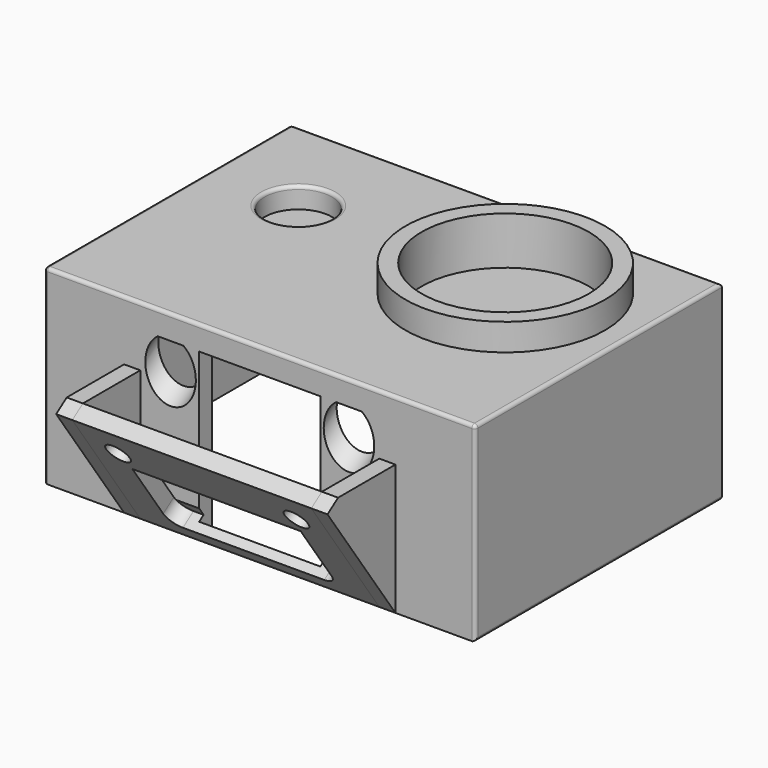
from build123d import *

# Parameters (mm, degrees)
F5_W         = 64
F5_H         = 45.8
F5_W_2       = 59.2
F5_H_2       = 41
F6_DEPTH     = 24.7
F7_W         = 64
F7_H         = 45.8
F7_W_2       = 59.2
F7_H_2       = 41
F8_DEPTH     = 3.6
F9_R         = 5
F10_DEPTH    = 3.1
F11_R        = 14.82
F11_R_2      = 12.42
F12_DEPTH    = 4
F13_DEPTH    = 3.1
F14_R        = 5
F15_DEPTH    = 2.4
F17_R        = 1.75
F18_DEPTH    = 2.4
F20_DEPTH    = 2.4
F22_DEPTH    = 2.4
F23_R        = 1.75
F24_REACH    = 60.9944299909
F25_R        = 0.5
F26_W        = 18
F26_H        = 2.4
F27_DEPTH    = 24.7
F28_R        = 3.75
F29_REACH    = 64.2512842404
F31_DEPTH    = 2.4
F32_T1_DEPTH = 2.4


# Not quite as in the source:
# - a fillet or chamfer that OpenCascade refuses, or shapes differently, is made with other operations: its cross-section is extruded or revolved along the edge and cut away or added
# - a feature names something its author has since deleted; it is built from what else it names


with BuildPart() as f6:
    # F5 (on Top) → F6 (new body)
    with BuildSketch(Plane.XY):
        Rectangle(F5_W, F5_H)
        Rectangle(F5_W_2, F5_H_2, mode=Mode.SUBTRACT)
    extrude(amount=F6_DEPTH)

    # F7 (on face) → F8 (join)
    with BuildSketch(Plane.XY.offset(24.7)):
        Rectangle(F7_W, F7_H)
        Rectangle(F7_W_2, F7_H_2, mode=Mode.SUBTRACT)
        Rectangle(F7_W_2, F7_H_2)
    extrude(amount=F8_DEPTH)

    # F9 (on face) → F10 (cut)
    with BuildSketch(Plane.XY.offset(28.3)):
        with Locations((-18.6, 7.5)):
            Circle(F9_R)
    extrude(amount=-F10_DEPTH, mode=Mode.SUBTRACT)

    # F11 (on face) → F12 (join)
    with BuildSketch(Plane.XY.offset(28.3)):
        with Locations((13.926, 5.264)):
            Circle(F11_R)
        with Locations((13.926, 5.264)):
            Circle(F11_R_2, mode=Mode.SUBTRACT)
    extrude(amount=F12_DEPTH)

    # F13 (cut): a face of the model
    f13_faces = [f6.faces().sort_by_distance(p)[0] for p in [
        (13.926, 5.264, 28.3),
    ]]
    extrude(f13_faces, amount=-F13_DEPTH, mode=Mode.SUBTRACT)

    # F14 (on face) → F15 (cut)
    with BuildSketch(Plane(origin=(0, 22.9, 0), x_dir=(-1, 0, 0), z_dir=(0, 1, 0))):
        with Locations((17.1, 14.15)):
            Circle(F14_R)
    extrude(amount=-F15_DEPTH, mode=Mode.SUBTRACT)

    # F17 (on face) → F18 (join)
    with BuildSketch(Plane(origin=(0, -15.3661306411, -10.759480508), x_dir=(-1, 0, 0), z_dir=(0, 0.8191520443, 0.5735764364))):
        Polygon((0, 24.1349003924), (0, 13.1349003924), (17.75, 13.1349003924), (17.75, 35.1349003924), (0, 35.1349003924), align=None)
        with Locations((13.25, 30.1349003924)):
            Circle(F17_R, mode=Mode.SUBTRACT)
        Polygon((-17.75, 13.1349003924), (0, 13.1349003924), (0, 24.1349003924), (0, 35.1349003924), (-17.75, 35.1349003924), align=None)
        with Locations((-13.25, 30.1349003924)):
            Circle(F17_R, mode=Mode.SUBTRACT)
    extrude(amount=F18_DEPTH)

    # F19 (on face) → F20 (join)
    with BuildSketch(Plane(origin=(-17.75, 0, 0), x_dir=(0, -1, 0), z_dir=(-1, 0, 0))):
        Polygon((22.9, 0), (35.5186815997, 18.0213449744), (33.5527166934, 19.3979284216), (22.9, 19.3979284216), align=None)
    extrude(amount=F20_DEPTH)

    # F21 (on face) → F22 (join)
    with BuildSketch(Plane.YZ.offset(17.75)):
        Polygon((-35.5186815997, 18.0213449744), (-22.9, 0), (-22.9, 19.3979284216), (-33.5527166934, 19.3979284216), align=None)
    extrude(amount=F22_DEPTH)

    f24_end = f6.faces().sort_by_distance((0, 0, 24.7))[0]
    # F23 (on face) → F24 (cut, up to a face of the model that its end follows)
    with BuildSketch(Plane(origin=(0, -15.3661306411, -10.759480508), x_dir=(1, 0, 0), z_dir=(0, -0.8191520443, -0.5735764364))):
        with Locations((-13.25, 30.1349003924)):
            Circle(F23_R)
        with Locations((13.25, 30.1349003924)):
            Circle(F23_R)
    f24_long = extrude(amount=-F24_REACH, mode=Mode.PRIVATE)
    add(split(f24_long, bisect_by=f24_end, keep=Keep.TOP, mode=Mode.PRIVATE), mode=Mode.SUBTRACT)

    # F25
    f25_edges = [f6.edges().sort_by_distance(p)[0] for p in [
        (-32, 0, 28.3),
        (0, -22.9, 28.3),
        (32, 0, 28.3),
        (0, 22.9, 28.3),
        (-23.6, 7.5, 28.3),
        (32, 0, 0),
        (0, 22.9, 0),
        (-32, 22.9, 14.15),
        (-32, 0, 0),
        (-32, -22.9, 14.15),
        (32, -22.9, 14.15),
    ]]
    fillet(f25_edges, radius=F25_R)

    # F26 (on face) → F27 (cut, through all)
    with BuildSketch(Plane(origin=(0, 0, 0), x_dir=(1, 0, 0), z_dir=(0, 0, -1))):
        with Locations((0, 21.7)):
            Rectangle(F26_W, F26_H)
    extrude(amount=-F27_DEPTH, mode=Mode.SUBTRACT)

    f29_end = Plane(origin=(0, -0.3794689119, 24.7), x_dir=(-1, 0, 0), z_dir=(0, 0, -1))
    # F28 (on face) → F29 (cut, up to a plane its end follows)
    with BuildSketch(Plane(origin=(0, -13.4001657348, -9.3828970608), x_dir=(-1, 0, 0), z_dir=(0, 0.8191520443, 0.5735764364))):
        with Locations((13.25, 30.1349003924)):
            Circle(F28_R)
        with Locations((-13.25, 30.1349003924)):
            Circle(F28_R)
    f29_long = extrude(amount=F29_REACH, mode=Mode.PRIVATE)
    add(split(f29_long, bisect_by=f29_end, keep=Keep.TOP, mode=Mode.PRIVATE), mode=Mode.SUBTRACT)

    # F30 (on face) → F31 (cut)
    with BuildSketch(Plane(origin=(0, -15.3661306411, -10.759480508), x_dir=(1, 0, 0), z_dir=(0, -0.8191520443, -0.5735764364))):
        Polygon((-12.5, 27.1349003924), (-12.5, 15.1349003924), (0, 15.1349003924), (12.5, 15.1349003924), (12.5, 27.1349003924), align=None)
    extrude(amount=-F31_DEPTH, mode=Mode.SUBTRACT)

    # F32: fillet of radius 2 on 2 edges, made by hand

    # F32_s2 → F32_t1 (join)
    with BuildSketch(Plane(origin=(0, -15.3661306411, -10.759480508), x_dir=(1, 0, 0), z_dir=(0, 0.8191520443, 0.5735764364))):
        with BuildLine():
            ThreePointArc((-10.5, -15.1349003924), (-11.9142135624, -15.7206868301), (-12.5, -17.1349003924))
            Line((-12.5, -17.1349003924), (-12.5, -15.1349003924))
            Line((-12.5, -15.1349003924), (-10.5, -15.1349003924))
        make_face()
        with BuildLine():
            ThreePointArc((12.5, -17.1349003924), (11.9142135624, -15.7206868301), (10.5, -15.1349003924))
            Line((10.5, -15.1349003924), (12.5, -15.1349003924))
            Line((12.5, -15.1349003924), (12.5, -17.1349003924))
        make_face()
    extrude(amount=F32_T1_DEPTH)


solid = f6.part
